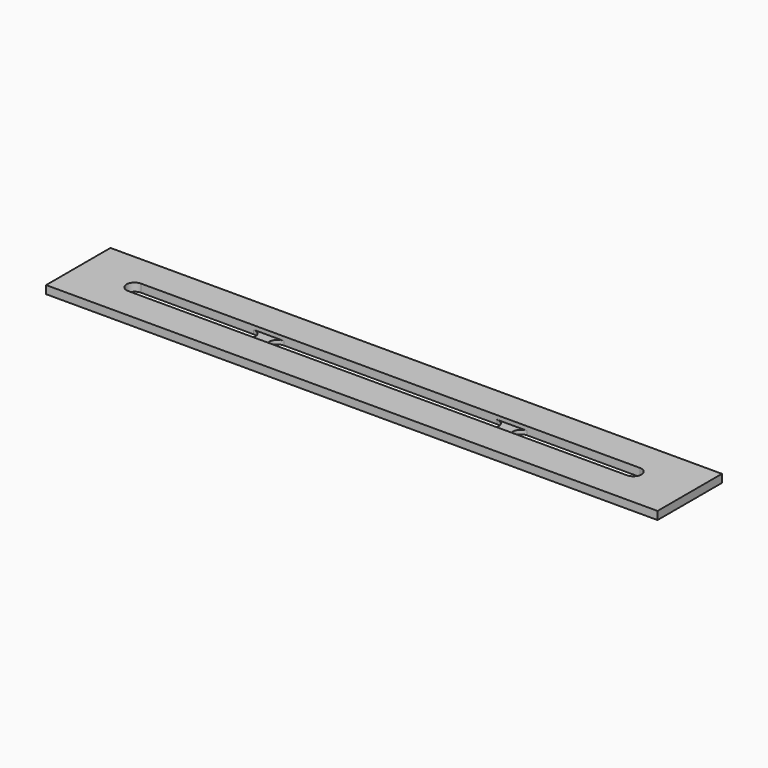
from build123d import *

# Parameters (mm, degrees)
F0_W     = 1930.4
F0_H     = 254
F1_DEPTH = 12.7
F3_DEPTH = 12.7


# Not quite as in the source:
# - ends of sketch curves that miss each other by under 0.0002 mm in the source are joined
# - a feature names something its author has since deleted; it is built from what else it names


with BuildPart() as f1:
    # F0 (on Top) → F1 (new body)
    with BuildSketch(Plane.XY):
        with Locations((-75.096349721, -133.9091630952)):
            Rectangle(F0_W, F0_H)
        with BuildLine():
            ThreePointArc((-862.496349721, -159.3091630952), (-887.896349721, -133.9091630952), (-862.496349721, -108.5091630952))
            Line((-862.496349721, -108.5091630952), (712.303650279, -108.5091630952))
            ThreePointArc((712.303650279, -108.5091630952), (737.703650279, -133.9091630952), (712.303650279, -159.3091630952))
            Line((712.303650279, -159.3091630952), (-862.496349721, -159.3091630952))
        make_face(mode=Mode.SUBTRACT)
    extrude(amount=F1_DEPTH)

    # F2 (on face) + F0 (on Top) → F3 (join)
    with BuildSketch(Plane(origin=(0, 0, 0), x_dir=(1, 0, 0), z_dir=(0, 0, -1))):
        with BuildLine():
            ThreePointArc((-506.896349721, 159.3091630952), (-481.496349721, 133.9091630952), (-506.896349721, 108.5091630952))
            Line((-506.896349721, 108.5091630952), (-411.646349721, 108.5091630952))
            ThreePointArc((-411.646349721, 108.5091630952), (-437.046349721, 133.9091630952), (-411.646349721, 159.3091630952))
            Line((-411.646349721, 159.3091630952), (-506.896349721, 159.3091630952))
        make_face()
        with BuildLine():
            ThreePointArc((261.453650279, 159.3091630952), (286.853650279, 133.9091630952), (261.453650279, 108.5091630952))
            Line((261.453650279, 108.5091630952), (356.703650279, 108.5091630952))
            ThreePointArc((356.703650279, 108.5091630952), (331.303650279, 133.9091630952), (356.703650279, 159.3091630952))
            Line((356.703650279, 159.3091630952), (261.453650279, 159.3091630952))
        make_face()
    with BuildSketch(Plane.XY):
        with Locations((-75.096349721, -133.9091630952)):
            Rectangle(F0_W, F0_H)
        with BuildLine():
            ThreePointArc((-862.496349721, -159.3091630952), (-887.896349721, -133.9091630952), (-862.496349721, -108.5091630952))
            Line((-862.496349721, -108.5091630952), (712.303650279, -108.5091630952))
            ThreePointArc((712.303650279, -108.5091630952), (737.703650279, -133.9091630952), (712.303650279, -159.3091630952))
            Line((712.303650279, -159.3091630952), (-862.496349721, -159.3091630952))
        make_face(mode=Mode.SUBTRACT)
    extrude(amount=F3_DEPTH, dir=(0, 0, -1))


solid = f1.part
